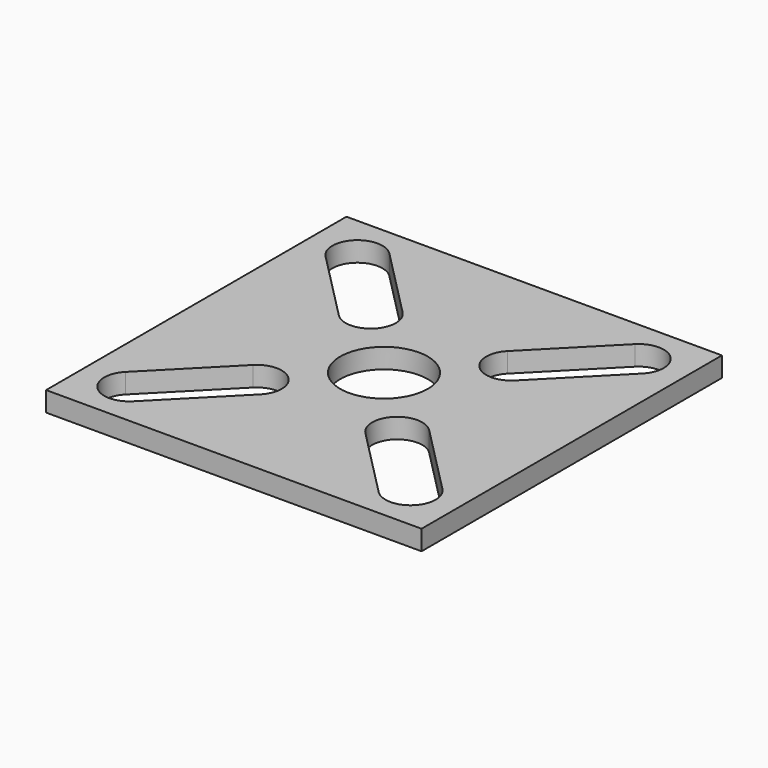
from build123d import *

# Parameters (mm, degrees)
F0_W     = 30
F0_H     = 30
F0_R     = 3.5
F1_DEPTH = 1.5875


# Not quite as in the source:
# - a length typed as a fraction of an inch, garbled in the dataset ("3 / 203.2 mm" for 3/8 in), is restored


with BuildPart() as f1:
    # F0 (on Top) → F1 (new body)
    with BuildSketch(Plane.XY):
        with Locations((-1.1622245609, -0.8481781135)):
            Rectangle(F0_W, F0_H)
        with BuildLine():
            Line((-13.8210662203, -10.8358568401), (-8.2036473316, -5.1398402471))
            ThreePointArc((-8.2036473316, -5.1398402471), (-5.3752884611, -5.120190821), (-5.355639035, -7.9485496914))
            Line((-5.355639035, -7.9485496914), (-10.9730579238, -13.6445662845))
            ThreePointArc((-10.9730579238, -13.6445662845), (-13.8014167942, -13.6642157105), (-13.8210662203, -10.8358568401))
        make_face(mode=Mode.SUBTRACT)
        with BuildLine():
            ThreePointArc((3.0311899132, -7.9485496914), (3.0508393392, -5.120190821), (5.8791982097, -5.1398402471))
            Line((5.8791982097, -5.1398402471), (11.4966170985, -10.8358568401))
            ThreePointArc((11.4966170985, -10.8358568401), (11.4769676724, -13.6642157105), (8.6486088019, -13.6445662845))
            Line((8.6486088019, -13.6445662845), (3.0311899132, -7.9485496914))
        make_face(mode=Mode.SUBTRACT)
        with Locations((-1.1622245609, -0.8481781135)):
            Circle(F0_R, mode=Mode.SUBTRACT)
        with BuildLine():
            ThreePointArc((-5.355639035, 6.2521934645), (-5.3752884611, 3.423834594), (-8.2036473316, 3.4434840201))
            Line((-8.2036473316, 3.4434840201), (-13.8210662203, 9.1395006131))
            ThreePointArc((-13.8210662203, 9.1395006131), (-13.8014167942, 11.9678594836), (-10.9730579238, 11.9482100575))
            Line((-10.9730579238, 11.9482100575), (-5.355639035, 6.2521934645))
        make_face(mode=Mode.SUBTRACT)
        with BuildLine():
            Line((3.0311899132, 6.2521934645), (8.6486088019, 11.9482100575))
            ThreePointArc((8.6486088019, 11.9482100575), (11.4769676724, 11.9678594836), (11.4966170985, 9.1395006131))
            Line((11.4966170985, 9.1395006131), (5.8791982097, 3.4434840201))
            ThreePointArc((5.8791982097, 3.4434840201), (3.0508393392, 3.423834594), (3.0311899132, 6.2521934645))
        make_face(mode=Mode.SUBTRACT)
    extrude(amount=F1_DEPTH)


solid = f1.part
